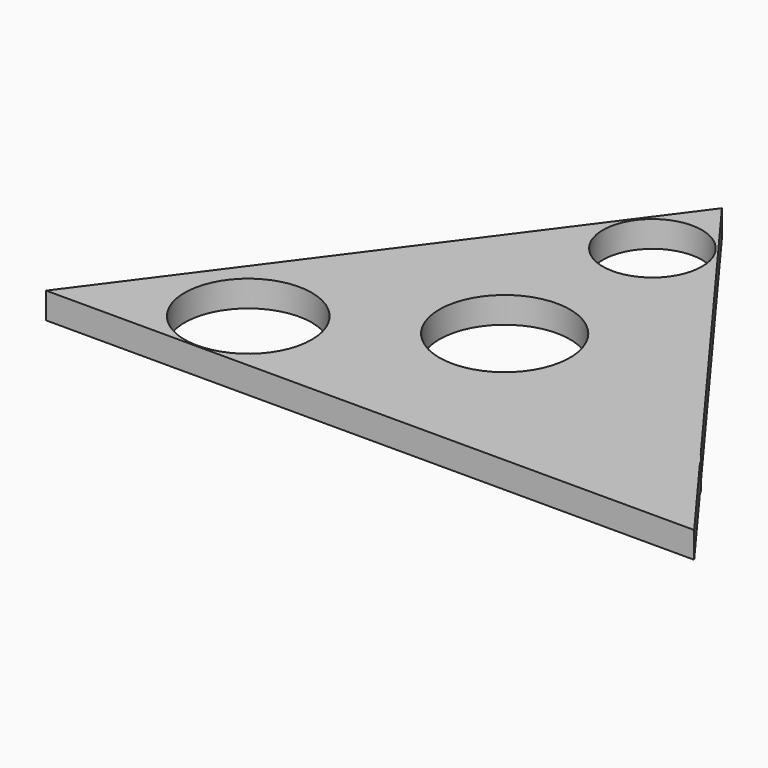
from build123d import *

# Parameters (mm, degrees)
F0_R     = 14.5320210998
F0_R_2   = 11.3186574679
F1_DEPTH = 6


# Not quite as in the source:
# - the program builds the solid bodies; features that only make, move or delete a surface that nothing else refers to are left out


with BuildPart() as f1:
    # F0 (on Top) → F1 (new body)
    with BuildSketch(Plane.XY):
        with BuildLine():
            Line((0, 62.0833449066), (-46.019215806, 0))
            Line((-46.019215806, 0), (-74.3083804846, -38.1641872227))
            Line((-74.3083804846, -38.1641872227), (73.8562121987, -38.1641872227))
            Line((73.8562121987, -38.1641872227), (58.8761133365, -17.8311929182))
            ThreePointArc((58.8761133365, -17.8311929182), (60.0804416969, -20.9630848338), (60.4900211693, -24.2934599519))
            ThreePointArc((60.4900211693, -24.2934599519), (34.0337461373, -29.5218920802), (56.5122905135, -14.6226963362))
            Line((56.5122905135, -14.6226963362), (0, 62.0833449066))
        make_face()
        with Locations((-39.9468056858, -23.3477279544)):
            Circle(F0_R, mode=Mode.SUBTRACT)
        with BuildLine():
            ThreePointArc((14.9293226936, 0), (0, -14.9293226936), (-14.9293226936, 0))
            ThreePointArc((-14.9293226936, 0), (0, 14.9293226936), (14.9293226936, 0))
        make_face(mode=Mode.SUBTRACT)
        with Locations((0, 42.2229841352)):
            Circle(F0_R_2, mode=Mode.SUBTRACT)
        with BuildLine():
            ThreePointArc((58.8761133365, -17.8311929182), (57.8111056109, -16.140817186), (56.5122905135, -14.6226963362))
            Line((56.5122905135, -14.6226963362), (58.8761133365, -17.8311929182))
        make_face()
        with BuildLine():
            Line((58.8761133365, -17.8311929182), (56.5122905135, -14.6226963362))
            ThreePointArc((56.5122905135, -14.6226963362), (34.0337461373, -29.5218920802), (60.4900211693, -24.2934599519))
            ThreePointArc((60.4900211693, -24.2934599519), (60.0804416969, -20.9630848338), (58.8761133365, -17.8311929182))
        make_face()
    extrude(amount=F1_DEPTH)


solid = f1.part
